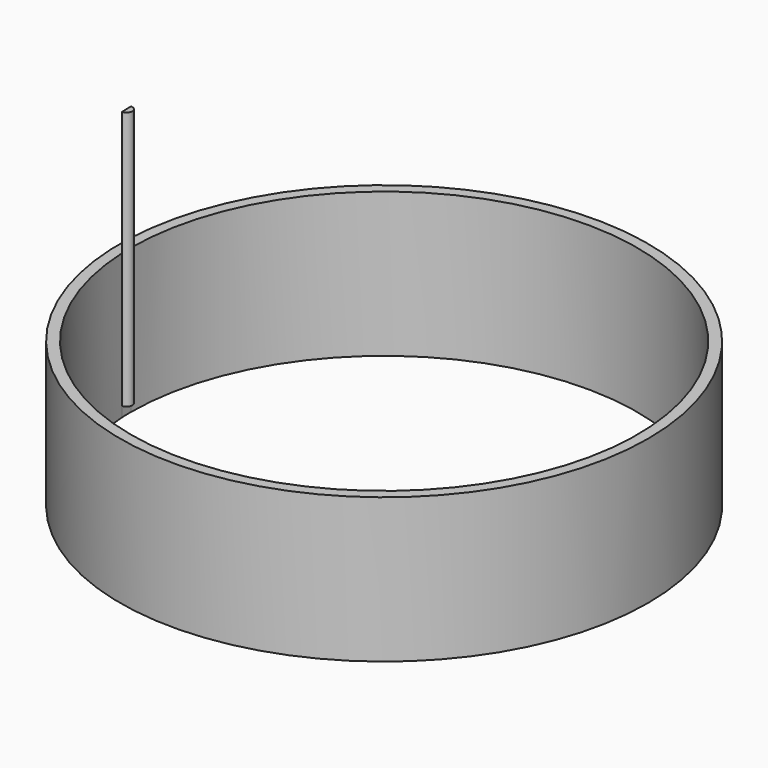
from build123d import *

# Parameters (mm, degrees)
F0_R          = 46.355
F1_DEPTH      = 25.4
F2_START      = 1.778
F2_DEPTH      = 21.844
F3_DEPTH      = 23.622
F3_DEPTH_BACK = 1.778


with BuildPart() as f1:
    # F0 (on Top) → F1 (new body)
    with BuildSketch(Plane.XY):
        Circle(F0_R)
        with BuildLine():
            ThreePointArc((-44.45, 0), (0, 44.45), (44.45, 0))
            ThreePointArc((44.45, 0), (1.016, -44.4383870544), (-44.4035542857, -2.0314691225))
            ThreePointArc((-44.4035542857, -2.0314691225), (-44.4383870544, -1.016), (-44.45, 0))
        make_face(mode=Mode.SUBTRACT)
    extrude(amount=F1_DEPTH)

    # F0 (on Top) → F2 (join)
    with BuildSketch(Plane.XY.offset(F2_START)):
        with BuildLine():
            ThreePointArc((-44.4035542857, -2.0314691225), (-43.4110425816, -0.9925117041), (-44.45, 0))
            ThreePointArc((-44.45, 0), (-44.4383870544, -1.016), (-44.4035542857, -2.0314691225))
        make_face()
    extrude(amount=F2_DEPTH)

    # F3 (add, two sides): a face of the model
    f3_faces = [f1.faces().sort_by_distance(p)[0] for p in [
        (-43.9998730556, -1.0059742036, 23.622),
    ]]
    extrude(f3_faces, amount=F3_DEPTH)
    extrude(f3_faces, amount=-F3_DEPTH_BACK)


solid = f1.part
